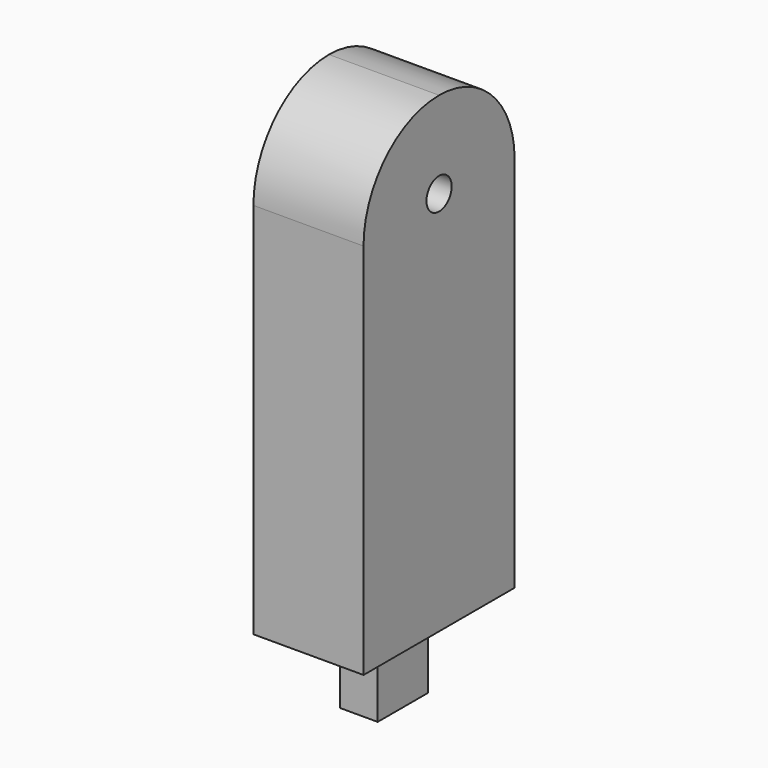
from build123d import *

# Parameters (mm, degrees)
F0_W     = 35
F0_H     = 60
F1_DEPTH = 150
F2_W     = 12
F2_H     = 20
F3_DEPTH = 25
F4_R     = 29.99999
F6_D     = 10


# Not quite as in the source:
# - a fillet or chamfer is up to 0.001 mm smaller than in the source, because OpenCascade refuses the exact size


with BuildPart() as f1:
    # F0 (on Top) → F1 (new body)
    with BuildSketch(Plane.XY):
        Rectangle(F0_W, F0_H)
    extrude(amount=F1_DEPTH)

    # F2 (on face) → F3 (join)
    with BuildSketch(Plane(origin=(0, 0, 0), x_dir=(1, 0, 0), z_dir=(0, 0, -1))):
        Rectangle(F2_W, F2_H)
    extrude(amount=F3_DEPTH)

    # F4 (radius 30 in the source; OpenCascade refuses exactly that, so slightly less here)
    f4_edges = [f1.edges().sort_by_distance(p)[0] for p in [
        (0, -30, 150),
        (0, 30, 150),
    ]]
    fillet(f4_edges, radius=F4_R)

    # F6 (through all)
    with Locations(Plane(origin=(-17.5, 0, 0), x_dir=(0, -1, 0), z_dir=(-1, 0, 0))):
        with Locations((0, 122.46029087)):
            Hole(F6_D / 2)


solid = f1.part
